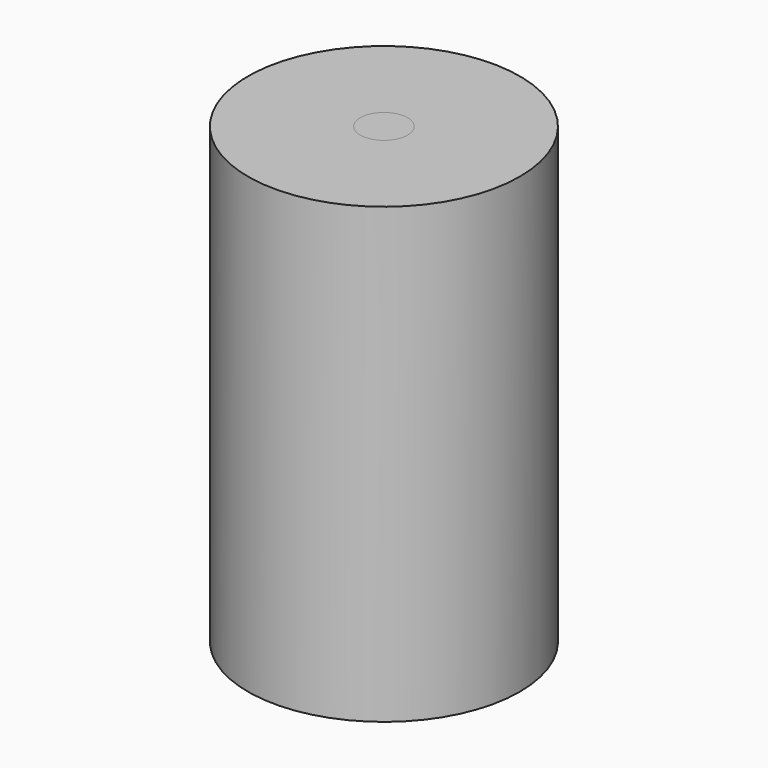
from build123d import *


with BuildPart() as f1:
    # F0 (on Front) → F1 (revolve)
    with BuildSketch(Plane.XZ):
        with BuildLine():
            add(Edge.make_bspline(
                [(2, 0), (2.0147597881, 4.0551168686), (6.1323122237, 11.3237550938), (16.688998986, 21.7541977077), (54.3363270254, 44.305808759), (64.9692962796, 90.6732568298), (30.4694363546, 98.7476745717), (10.6389869017, 99.7502924966)],
                knots=[0, 0, 0, 0, 0.1227515264, 0.2623319068, 0.5034894894, 0.723265145, 0.9584765665, 0.9584765665, 0.9584765665, 0.9584765665], degree=3))
            Line((2, 0), (61.1463077366, 0))
            Line((61.1463077366, 0), (61.1463077366, 102))
            Line((61.1463077366, 102), (10.6389869017, 102))
            Line((10.6389869017, 102), (10.6389869017, 99.7502924966))
        make_face()
        with BuildLine():
            Line((61.1463077366, 0), (2, 0))
            add(Edge.make_bspline(
                [(2, 0), (2.0147597881, -4.0551168686), (6.1323122237, -11.3237550938), (16.688998986, -21.7541977077), (54.3363270254, -44.305808759), (65.6035285267, -93.4389688412), (23.8270945847, -100.0363081694), (0, -100)],
                knots=[0, 0, 0, 0, 0.1227515264, 0.2623319068, 0.5034894894, 0.723265145, 1, 1, 1, 1], degree=3))
            Line((0, -100), (0, -102))
            Line((0, -102), (61.1463077366, -102))
            Line((61.1463077366, -102), (61.1463077366, 0))
        make_face()
    revolve(axis=Axis((0, 0, 50), (0, 0, 1)))


with BuildPart() as f2:
    # F0 (on Front) → F2 (revolve)
    with BuildSketch(Plane.XZ):
        with BuildLine():
            add(Edge.make_bspline(
                [(10.6389869017, 99.7502924966), (7.1381860311, 99.9272912939), (3.5752011705, 100.005447958), (0, 100)],
                knots=[0.9584765665, 0.9584765665, 0.9584765665, 0.9584765665, 1, 1, 1, 1], degree=3))
            Line((10.6389869017, 99.7502924966), (10.6389869017, 102))
            Line((10.6389869017, 102), (0, 102))
            Line((0, 102), (0, 100))
        make_face()
    revolve(axis=Axis((0, 0, 50), (0, 0, 1)))


with BuildPart() as f3:
    # F0 (on Front) → F3 (revolve)
    with BuildSketch(Plane.XZ):
        with BuildLine():
            Line((0, 99.618345499), (0, 15.0721119717))
            add(Edge.make_bspline(
                [(0, 99.618345499), (1.3623338784, 99.5932547672), (4.3850885304, 99.5375832996), (10.8135018916, 99.3072595025), (18.7031980542, 98.7158812691), (27.9486517628, 97.61722578), (38.1496670262, 94.8631175555), (46.5191243788, 91.7482221565), (55.3848555365, 84.7315803035), (57.8540814168, 75.1230097649), (57.5917895539, 67.7529895608), (54.6124455282, 58.9976189554), (47.1400496162, 46.1868707392), (37.1177594466, 37.4951198572), (26.4708786817, 28.8302422015), (15.9709875668, 21.2931010192), (6.5001510156, 15.6502063645), (1.9614894282, 15.2465580787), (0, 15.0721119717)],
                knots=[0, 0, 0, 0, 0.041916508, 0.0930046015, 0.1501329622, 0.2122987352, 0.277831124, 0.3387369607, 0.4053335032, 0.4677200062, 0.5217235792, 0.5827014437, 0.6602929687, 0.7345452588, 0.8093922215, 0.8831321428, 0.9494928049, 1, 1, 1, 1], degree=3))
        make_face()
    revolve(axis=Axis((0, 0, 50), (0, 0, 1)))


solid = Compound([f1.part, f2.part, f3.part])
